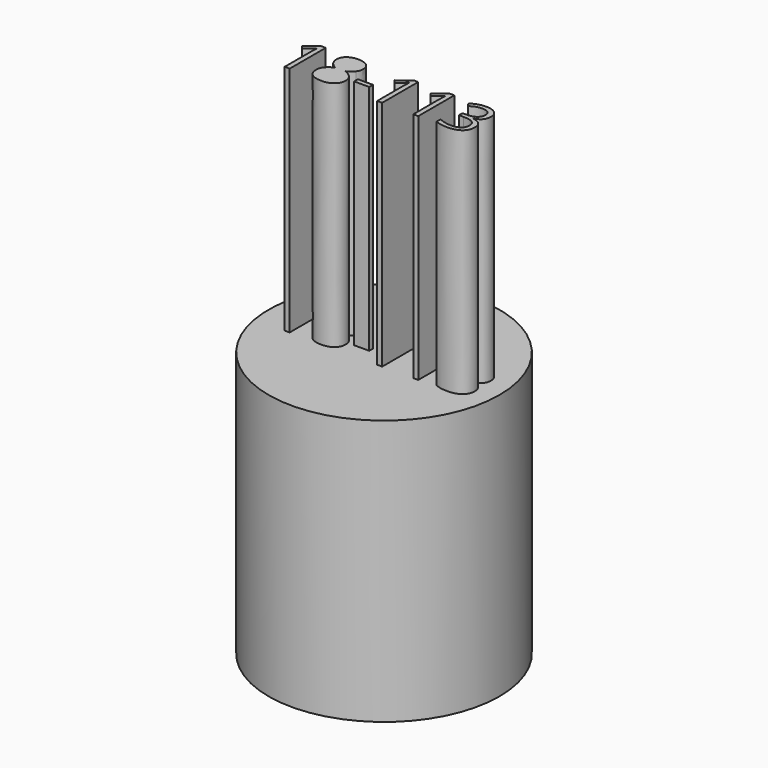
from build123d import *

# Parameters (mm, degrees)
F0_R         = 65.6596239796
F1_DEPTH     = 150.876
F2_TEXT_SIZE = 35.8965285761
F4_DEPTH     = 132.08


# Not quite as in the source:
# - Text() gives the source's letters only with a copy of the font that has no kerning and outlines rounded to 1/6400 em; it was checked with that copy


with BuildPart() as f1:
    # F0 (on Top) → F1 (new body)
    with BuildSketch(Plane.XY):
        Circle(F0_R)
    extrude(amount=F1_DEPTH)

    # F3 (on face) + F2 (on face) → F4 (join)
    with BuildSketch(Plane.XY.offset(150.876)):
        with BuildLine():
            add(Edge.make_bspline(
                [(-31.9479104328, 13.09928544), (-29.8894688722, 14.7538910541), (-26.4344279968, 14.7538910541)],
                knots=[0, 0, 0, 1, 1, 1], degree=2))
            add(Edge.make_bspline(
                [(-34.0063519933, 8.6570900288), (-34.0063519933, 11.444679826), (-31.9479104328, 13.09928544)],
                knots=[0, 0, 0, 1, 1, 1], degree=2))
            add(Edge.make_bspline(
                [(-32.9546958827, 5.1066989993), (-34.0063519933, 6.6939986222), (-34.0063519933, 8.6570900288)],
                knots=[0, 0, 0, 1, 1, 1], degree=2))
            add(Edge.make_bspline(
                [(-29.4856329257, 2.1564530569), (-31.903039772, 3.5193993763), (-32.9546958827, 5.1066989993)],
                knots=[0, 0, 0, 1, 1, 1], degree=2))
            add(Edge.make_bspline(
                [(-34.8476768818, -4.6975403681), (-34.8476768818, -0.3002156175), (-29.4856329257, 2.1564530569)],
                knots=[0, 0, 0, 1, 1, 1], degree=2))
            add(Edge.make_bspline(
                [(-32.6377968413, -9.7931647761), (-34.8476768818, -7.995533931), (-34.8476768818, -4.6975403681)],
                knots=[0, 0, 0, 1, 1, 1], degree=2))
            add(Edge.make_bspline(
                [(-26.3278601776, -11.5907956212), (-30.4279168009, -11.5907956212), (-32.6377968413, -9.7931647761)],
                knots=[0, 0, 0, 1, 1, 1], degree=2))
            add(Edge.make_bspline(
                [(-20.2310591522, -9.6865969569), (-22.4577656904, -11.5907956212), (-26.3278601776, -11.5907956212)],
                knots=[0, 0, 0, 1, 1, 1], degree=2))
            add(Edge.make_bspline(
                [(-18.004352614, -4.5965813815), (-18.004352614, -7.7823982926), (-20.2310591522, -9.6865969569)],
                knots=[0, 0, 0, 1, 1, 1], degree=2))
            add(Edge.make_bspline(
                [(-19.3196238563, -0.799401718), (-18.004352614, -2.4371808343), (-18.004352614, -4.5965813815)],
                knots=[0, 0, 0, 1, 1, 1], degree=2))
            add(Edge.make_bspline(
                [(-23.7534060187, 2.3303268672), (-20.6348950987, 0.8383773983), (-19.3196238563, -0.799401718)],
                knots=[0, 0, 0, 1, 1, 1], degree=2))
            add(Edge.make_bspline(
                [(-20.001097016, 5.1683961578), (-21.1733430273, 3.6091406977), (-23.7534060187, 2.3303268672)],
                knots=[0, 0, 0, 1, 1, 1], degree=2))
            add(Edge.make_bspline(
                [(-18.8288510047, 8.6234370332), (-18.8288510047, 6.7276516178), (-20.001097016, 5.1683961578)],
                knots=[0, 0, 0, 1, 1, 1], degree=2))
            add(Edge.make_bspline(
                [(-20.8788793163, 13.1245251867), (-18.8288510047, 11.4951593193), (-18.8288510047, 8.6234370332)],
                knots=[0, 0, 0, 1, 1, 1], degree=2))
            add(Edge.make_bspline(
                [(-26.4344279968, 14.7538910541), (-22.928907628, 14.7538910541), (-20.8788793163, 13.1245251867)],
                knots=[0, 0, 0, 1, 1, 1], degree=2))
        make_face()
    with BuildSketch(Plane.XY.offset(150.876)):
        with Locations((-57.1932659204, -11.237439168)):
            Text('18-113', F2_TEXT_SIZE, font='Open Sans', text_align=(TextAlign.LEFT, TextAlign.BOTTOM))
    extrude(amount=F4_DEPTH)


solid = f1.part
